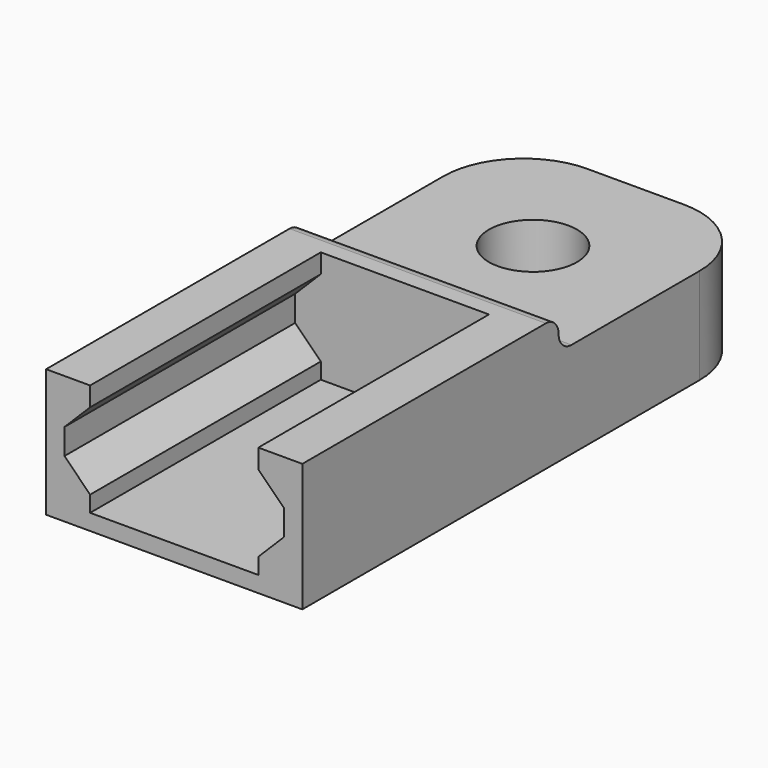
from build123d import *

# Parameters (mm, degrees)
F1_DEPTH = 9
F3_DEPTH = 2
F4_W     = 16
F4_H     = 16
F5_DEPTH = 6
F6_D     = 5.5
F7_R     = 5
F8_R     = 0.99999


# Not quite as in the source:
# - a fillet or chamfer is up to 0.001 mm smaller than in the source, because OpenCascade refuses the exact size


with BuildPart() as f1:
    # F0 (on Front) → F1 (new body, symmetric)
    with BuildSketch(Plane.XZ):
        Polygon((-6.85, -0.8), (-6.85, 0.8), (-5.25, 2.4), (-5.25, 3.6), (-8, 3.6), (-8, -4.4), (0, -4.4), (8, -4.4), (8, 3.6), (5.25, 3.6), (5.25, 2.4), (6.85, 0.8), (6.85, -0.8), (5.25, -2.4), (5.25, -3.4), (0, -3.4), (-5.25, -3.4), (-5.25, -2.4), align=None)
    extrude(amount=F1_DEPTH, both=True)

    # F2 (on face) → F3 (join)
    with BuildSketch(Plane(origin=(0, 9, 0), x_dir=(-1, 0, 0), z_dir=(0, 1, 0))):
        Polygon((-5.25, 2.4), (-5.25, 3.6), (-8, 3.6), (-8, -4.4), (8, -4.4), (8, 3.6), (5.25, 3.6), (5.25, 2.4), (6.85, 0.8), (6.85, -0.8), (5.25, -2.4), (5.25, -3.4), (-5.25, -3.4), (-5.25, -2.4), (-6.85, -0.8), (-6.85, 0.8), align=None)
        Polygon((5.25, 3.6), (-5.25, 3.6), (-5.25, 2.4), (-6.85, 0.8), (-6.85, -0.8), (-5.25, -2.4), (-5.25, -3.4), (5.25, -3.4), (5.25, -2.4), (6.85, -0.8), (6.85, 0.8), (5.25, 2.4), align=None)
    extrude(amount=F3_DEPTH)

    # F4 (on face) → F5 (join)
    with BuildSketch(Plane(origin=(0, 0, -4.4), x_dir=(1, 0, 0), z_dir=(0, 0, -1))):
        with Locations((0, -19)):
            Rectangle(F4_W, F4_H)
    extrude(amount=-F5_DEPTH)

    # F6 (through all)
    with Locations(Plane(origin=(0, 0, -4.4), x_dir=(1, 0, 0), z_dir=(0, 0, -1))):
        with Locations((0, -19)):
            Hole(F6_D / 2)

    # F7
    f7_edges = [f1.edges().sort_by_distance(p)[0] for p in [
        (8, 27, -1.4),
        (-8, 27, -1.4),
    ]]
    fillet(f7_edges, radius=F7_R)

    # F8 (radius 1 in the source; OpenCascade refuses exactly that, so slightly less here)
    f8_edges = [f1.edges().sort_by_distance(p)[0] for p in [
        (0, 11, 1.6),
        (0, 11, 3.6),
    ]]
    fillet(f8_edges, radius=F8_R)


solid = f1.part
